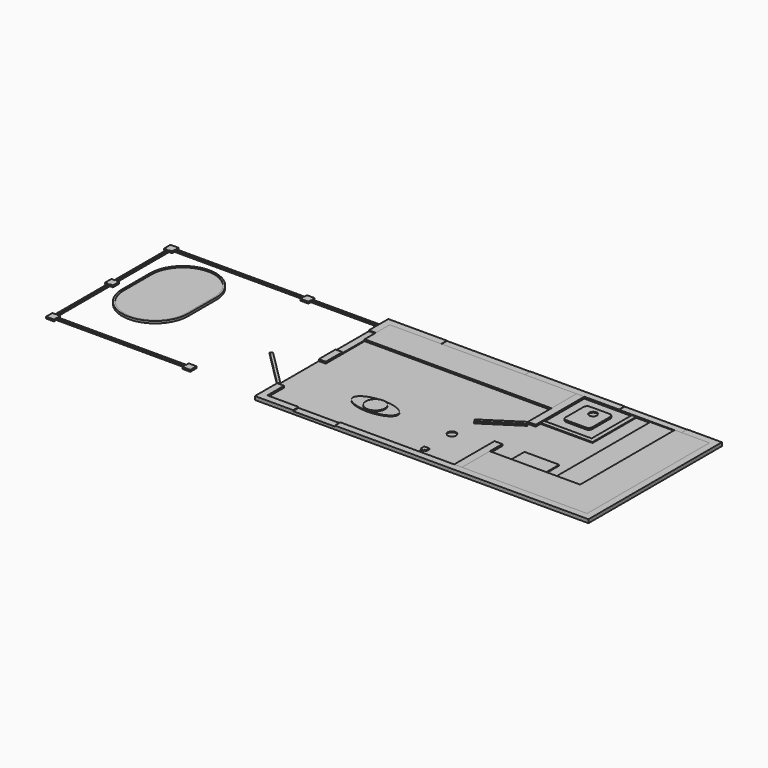
from build123d import *

# Parameters (mm, degrees)
F0_W      = 4876.8
F0_H      = 2438.4
F1_DEPTH  = 25.4
F2_W      = 4876.8
F2_H      = 2438.4
F2_W_2    = 4673.6
F2_H_2    = 2235.2
F3_DEPTH  = 25.4
F4_W      = 114.3
F4_H      = 2235.2
F5_DEPTH  = 25.4
F6_W      = 114.3
F6_H      = 609.6
F7_DEPTH  = 25.4
F8_W      = 101.6
F8_H      = 762
F9_DEPTH  = 25.4
F11_DEPTH = 25.4
F13_DEPTH = 25.4
F14_W     = 355.6
F14_H     = 1727.2
F15_DEPTH = 12.7
F17_DEPTH = 25.4
F19_DEPTH = 25.4
F20_R     = 63.5
F21_DEPTH = 12.7
F23_DEPTH = 12.7
F24_W     = 2730.5
F24_H     = 457.2
F25_DEPTH = 25.4
F26_W     = 609.6
F26_H     = 101.6
F26_W_2   = 101.6
F26_H_2   = 609.6
F27_DEPTH = 12.7
F28_R     = 57.5
F29_DEPTH = 12.7
F31_DEPTH = 25.4
F30_W     = 1879.6
F30_H     = 25.4
F32_DEPTH = 25.4
F30_W_2   = 25.4
F30_H_2   = 965.2
F30_W_3   = 1009.65
F33_R     = 139.7
F34_DEPTH = 25.4
F35_DEPTH = 12.7
F37_DEPTH = 25.4
F39_DEPTH = 6.35
F40_W     = 1219.2
F40_H     = 101.6
F40_W_2   = 914.4
F41_DEPTH = 3.175
F42_W     = 508
F42_H     = 254
F43_DEPTH = 12.7
F45_DEPTH = 12.7


# Not quite as in the source:
# - a feature names something its author has since deleted; it is built from what else it names


with BuildPart() as f1:
    # F0 (on Top) → F1 (new body)
    with BuildSketch(Plane.XY):
        Rectangle(F0_W, F0_H)
    extrude(amount=F1_DEPTH)

    # F20 (on face) → F21 (cut)
    with BuildSketch(Plane.XY.offset(25.4)):
        with Locations((-127, -508)):
            Circle(F20_R)
    extrude(amount=-F21_DEPTH, mode=Mode.SUBTRACT)

    # F33 (on face) → F34 (join)
    with BuildSketch(Plane.XY.offset(25.4)):
        with Locations((-1228.4452915192, -528.5891890526)):
            Circle(F33_R)
    extrude(amount=F34_DEPTH)

    # F33 (on face) → F35 (join)
    with BuildSketch(Plane.XY.offset(25.4)):
        with BuildLine():
            add(Edge.make_bspline(
                [(-1558.6452915192, -528.5891890526), (-1558.6452915192, -792.5537321261), (-1063.3452915192, -660.5714605893), (-568.0452915192, -528.5891890526), (-1063.3452915192, -396.6069175158), (-1558.6452915192, -264.6246459791), (-1558.6452915192, -528.5891890526)],
                knots=[0, 0, 0, 2.0943951024, 2.0943951024, 4.1887902048, 4.1887902048, 6.2831853072, 6.2831853072, 6.2831853072], degree=2, weights=[1, 0.5, 1, 0.5, 1, 0.5, 1]))
        make_face()
        with Locations((-1228.4452915192, -528.5891890526)):
            Circle(F33_R, mode=Mode.SUBTRACT)
    extrude(amount=F35_DEPTH)


with BuildPart() as f3:
    # F2 (on face) → F3 (new body)
    with BuildSketch(Plane.XY.offset(25.4)):
        Rectangle(F2_W, F2_H)
        Rectangle(F2_W_2, F2_H_2, mode=Mode.SUBTRACT)
    extrude(amount=F3_DEPTH)

    # F8 (on face) → F9 (cut)
    with BuildSketch(Plane.XY.offset(50.8)):
        with Locations((-2387.6, -431.8)):
            Rectangle(F8_W, F8_H)
    extrude(amount=-F9_DEPTH, mode=Mode.SUBTRACT)

    # F26 (on face) → F27 (cut)
    with BuildSketch(Plane.XY.offset(50.8)):
        with Locations((-1574.8, -1168.4)):
            Rectangle(F26_W, F26_H)
        with Locations((-2387.6, 558.8)):
            Rectangle(F26_W_2, F26_H_2)
    extrude(amount=-F27_DEPTH, mode=Mode.SUBTRACT)

    # F40 (on face) → F41 (cut)
    with BuildSketch(Plane.XY.offset(50.8)):
        with Locations((-971.55, 1168.4)):
            Rectangle(F40_W, F40_H)
        with Locations((1473.2, 1168.4)):
            Rectangle(F40_W_2, F40_H)
    extrude(amount=-F41_DEPTH, mode=Mode.SUBTRACT)


with BuildPart() as f5:
    # F4 (on face) → F5 (new body)
    with BuildSketch(Plane.XY.offset(25.4)):
        with Locations((450.85, 0)):
            Rectangle(F4_W, F4_H)
    extrude(amount=F5_DEPTH)

    # F6 (on face) → F7 (cut)
    with BuildSketch(Plane.XY.offset(50.8)):
        with Locations((450.85, -76.2)):
            Rectangle(F6_W, F6_H)
    extrude(amount=-F7_DEPTH, mode=Mode.SUBTRACT)


with BuildPart() as f11:
    # F10 (on face) → F11 (new body)
    with BuildSketch(Plane.XY.offset(25.4)):
        with BuildLine():
            Line((999.6, 965.2), (711.2, 965.2))
            ThreePointArc((711.2, 965.2), (675.2789755157, 950.3210244843), (660.4, 914.4))
            Line((660.4, 914.4), (660.4, 586))
            ThreePointArc((660.4, 586), (675.2789755157, 550.0789755157), (711.2, 535.2))
            Line((711.2, 535.2), (999.6, 535.2))
            ThreePointArc((999.6, 535.2), (1035.5210244843, 550.0789755157), (1050.4, 586))
            Line((1050.4, 586), (1050.4, 914.4))
            ThreePointArc((1050.4, 914.4), (1035.5210244843, 950.3210244843), (999.6, 965.2))
        make_face()
    extrude(amount=F11_DEPTH)

    # F28 (on face) → F29 (cut)
    with BuildSketch(Plane.XY.offset(50.8)):
        with Locations((855.4, 845.2)):
            Circle(F28_R)
    extrude(amount=-F29_DEPTH, mode=Mode.SUBTRACT)


with BuildPart() as f13:
    # F12 (on face) → F13 (new body)
    with BuildSketch(Plane.XY.offset(25.4)):
        Polygon((508, -609.6), (508, -1117.6), (2336.8, -1117.6), (2336.8, 1117.6), (1828.8, 1117.6), (1828.8, -609.6), align=None)
    extrude(amount=F13_DEPTH)


with BuildPart() as f15:
    # F14 (on face) → F15 (new body)
    with BuildSketch(Plane.XY.offset(25.4)):
        with Locations((1651, 254)):
            Rectangle(F14_W, F14_H)
    extrude(amount=F15_DEPTH)


with BuildPart() as f17:
    # F16 (on face) → F17 (new body)
    with BuildSketch(Plane.XY.offset(25.4)):
        Polygon((421.3120895758, 185.9594968457), (393.7, 228.6), (-117.9860378521, -102.7450749101), (-90.3739482763, -145.3855780644), align=None)
    extrude(amount=F17_DEPTH)


with BuildPart() as f19:
    # F18 (on face) → F19 (new body)
    with BuildSketch(Plane.XY.offset(25.4)):
        Polygon((-2438.4, -812.8), (-2411.4592316368, -785.8592316368), (-2950.2745989009, -247.0438643726), (-2977.2153672641, -273.9846327359), align=None)
    extrude(amount=F19_DEPTH)


with BuildPart() as f23:
    # F22 (on face) → F23 (new body)
    with BuildSketch(Plane.XY.offset(25.4)):
        with BuildLine():
            Line((-139.7, -1028.7), (-139.7, -1117.6))
            Line((-139.7, -1117.6), (-114.3, -1117.6))
            Line((-114.3, -1117.6), (-114.3, -1028.7))
            Line((-114.3, -1028.7), (-95.25, -1028.7))
            ThreePointArc((-95.25, -1028.7), (-90.7598719395, -1026.8401280605), (-88.9, -1022.35))
            Line((-88.9, -1022.35), (-88.9, -971.55))
            ThreePointArc((-88.9, -971.55), (-90.7598719395, -967.0598719395), (-95.25, -965.2))
            Line((-95.25, -965.2), (-158.75, -965.2))
            ThreePointArc((-158.75, -965.2), (-163.2401280605, -967.0598719395), (-165.1, -971.55))
            Line((-165.1, -971.55), (-165.1, -1022.35))
            ThreePointArc((-165.1, -1022.35), (-163.2401280605, -1026.8401280605), (-158.75, -1028.7))
            Line((-158.75, -1028.7), (-139.7, -1028.7))
        make_face()
    extrude(amount=F23_DEPTH)


with BuildPart() as f25:
    # F24 (on face) → F25 (new body)
    with BuildSketch(Plane.XY.offset(25.4)):
        with Locations((-971.55, 889)):
            Rectangle(F24_W, F24_H)
    extrude(amount=F25_DEPTH)


with BuildPart() as f31:
    # F30 (on Top) → F31 (new body)
    with BuildSketch(Plane.XY):
        Polygon((-5441.95, -1022.35), (-5486.4, -1022.35), (-5511.8, -1022.35), (-5556.25, -1022.35), (-5556.25, -1136.65), (-5441.95, -1136.65), (-5441.95, -1092.2), (-5441.95, -1066.8), align=None)
    extrude(amount=F31_DEPTH)


with BuildPart() as f31b:
    # F30 (on Top) → F31, piece 2 (new body)
    with BuildSketch(Plane.XY):
        Polygon((-3562.35, -1022.35), (-3562.35, -1066.8), (-3562.35, -1092.2), (-3562.35, -1136.65), (-3448.05, -1136.65), (-3448.05, -1022.35), align=None)
    extrude(amount=F31_DEPTH)


with BuildPart() as f31c:
    # F30 (on Top) → F31, piece 3 (new body)
    with BuildSketch(Plane.XY):
        Polygon((-5441.95, 57.15), (-5486.4, 57.15), (-5511.8, 57.15), (-5556.25, 57.15), (-5556.25, -57.15), (-5511.8, -57.15), (-5486.4, -57.15), (-5441.95, -57.15), align=None)
    extrude(amount=F31_DEPTH)


with BuildPart() as f31d:
    # F30 (on Top) → F31, piece 4 (new body)
    with BuildSketch(Plane.XY):
        Polygon((-5486.4, 1022.35), (-5441.95, 1022.35), (-5441.95, 1066.8), (-5441.95, 1092.2), (-5441.95, 1136.65), (-5556.25, 1136.65), (-5556.25, 1022.35), (-5511.8, 1022.35), align=None)
    extrude(amount=F31_DEPTH)


with BuildPart() as f32:
    # F30 (on Top) → F32 (new body)
    with BuildSketch(Plane.XY):
        with Locations((-4502.15, -1079.5)):
            Rectangle(F30_W, F30_H)
    extrude(amount=F32_DEPTH)


with BuildPart() as f32b:
    # F30 (on Top) → F32, piece 2 (new body)
    with BuildSketch(Plane.XY):
        with Locations((-5499.1, -539.75)):
            Rectangle(F30_W_2, F30_H_2)
    extrude(amount=F32_DEPTH)


with BuildPart() as f32c:
    # F30 (on Top) → F32, piece 3 (new body)
    with BuildSketch(Plane.XY):
        with Locations((-5499.1, 539.75)):
            Rectangle(F30_W_2, F30_H_2)
    extrude(amount=F32_DEPTH)


with BuildPart() as f32d:
    # F30 (on Top) → F32, piece 4 (new body)
    with BuildSketch(Plane.XY):
        with Locations((-4502.15, 1079.5)):
            Rectangle(F30_W, F30_H)
        Polygon((-3562.35, 1092.2), (-3562.35, 1066.8), (-3562.35, 1022.35), (-3448.05, 1022.35), (-3448.05, 1066.8), (-3448.05, 1092.2), (-3448.05, 1136.65), (-3562.35, 1136.65), align=None)
        with Locations((-2943.225, 1079.5)):
            Rectangle(F30_W_3, F30_H)
    extrude(amount=F32_DEPTH)


with BuildPart() as f37:
    # F36 (on Top) → F37 (new body)
    with BuildSketch(Plane.XY):
        with BuildLine():
            ThreePointArc((-4809.5684051514, 913.8274442911), (-5150.818137752, 772.4771768917), (-5292.1684051514, 431.2274442911))
            Line((-5292.1684051514, 431.2274442911), (-5292.1684051514, -76.7725557089))
            ThreePointArc((-5292.1684051514, -76.7725557089), (-5150.818137752, -418.0222883095), (-4809.5684051514, -559.3725557089))
            ThreePointArc((-4809.5684051514, -559.3725557089), (-4468.3186725507, -418.0222883095), (-4326.9684051514, -76.7725557089))
            Line((-4326.9684051514, -76.7725557089), (-4326.9684051514, 431.2274442911))
            ThreePointArc((-4326.9684051514, 431.2274442911), (-4468.3186725507, 772.4771768917), (-4809.5684051514, 913.8274442911))
        make_face()
    extrude(amount=F37_DEPTH)

    # F38 (on face) → F39 (join)
    with BuildSketch(Plane.XY.offset(25.4)):
        with BuildLine():
            Line((-4326.9684051514, -76.7725557089), (-4326.9684051514, 431.2274442911))
            ThreePointArc((-4326.9684051514, 431.2274442911), (-4809.5684051514, 913.8274442911), (-5292.1684051514, 431.2274442911))
            Line((-5292.1684051514, 431.2274442911), (-5292.1684051514, -76.7725557089))
            ThreePointArc((-5292.1684051514, -76.7725557089), (-4809.5684051514, -559.3725557089), (-4326.9684051514, -76.7725557089))
        make_face()
        with BuildLine():
            ThreePointArc((-5266.7684051514, 431.2274442911), (-4809.5684051514, 888.4274442911), (-4352.3684051514, 431.2274442911))
            Line((-4352.3684051514, 431.2274442911), (-4352.3684051514, -76.7725557089))
            ThreePointArc((-4352.3684051514, -76.7725557089), (-4809.5684051514, -533.9725557089), (-5266.7684051514, -76.7725557089))
            Line((-5266.7684051514, -76.7725557089), (-5266.7684051514, 431.2274442911))
        make_face(mode=Mode.SUBTRACT)
    extrude(amount=F39_DEPTH)


with BuildPart() as f43:
    # F42 (on face) → F43 (new body)
    with BuildSketch(Plane.XY.offset(25.4)):
        with Locations((1065.4114627128, -482.6)):
            Rectangle(F42_W, F42_H)
    extrude(amount=F43_DEPTH)


with BuildPart() as f45:
    # F44 (on face) → F45 (new body)
    with BuildSketch(Plane.XY.offset(25.4)):
        Polygon((1202.8, 382.8), (508, 382.8), (508, 319.3), (1266.3, 319.3), (1266.3, 1117.6), (1202.8, 1117.6), align=None)
    extrude(amount=F45_DEPTH)


solid = Compound([f1.part, f3.part, f5.part, f11.part, f13.part, f15.part, f17.part, f19.part, f23.part, f25.part, f31.part, f31b.part, f31c.part, f31d.part, f32.part, f32b.part, f32c.part, f32d.part, f37.part, f43.part, f45.part])
